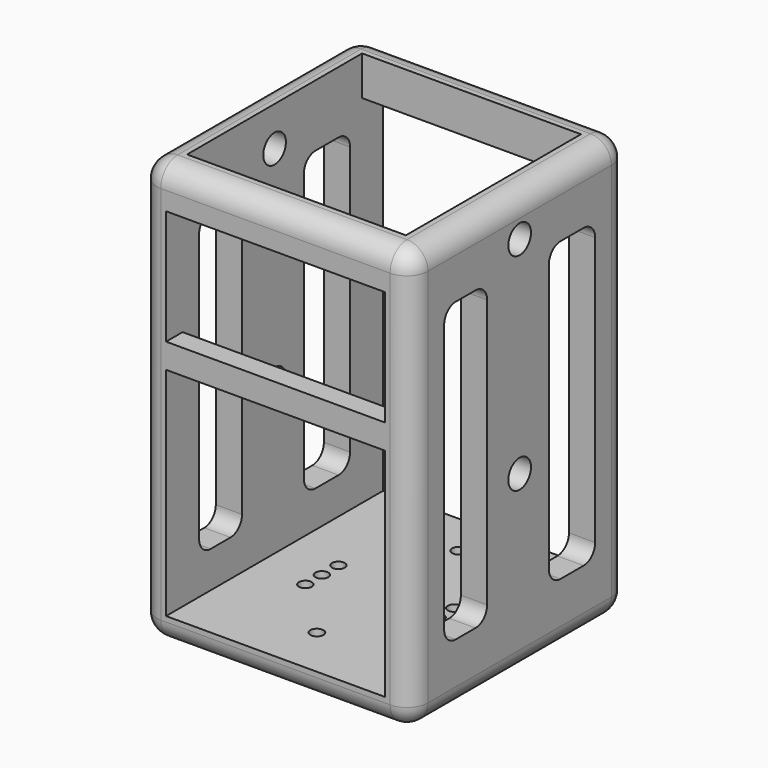
from build123d import *

# Parameters (mm, degrees)
F0_W      = 65.7
F0_H      = 65.7
F1_DEPTH  = 3.175
F2_W      = 65.7
F2_H      = 99
F2_W_2    = 53
F2_H_2    = 86.3
F3_DEPTH  = 65.7
F4_DEPTH  = 6.35
F5_R      = 3.429
F6_DEPTH  = 65.701
F7_R      = 5.08
F8_W      = 53
F8_H      = 6
F9_DEPTH  = 5
F10_R     = 1.5875
F10_R_2   = 1.55
F11_DEPTH = 10


# Not quite as in the source:
# - a length typed as a fraction of an inch, garbled in the dataset ("3 / 203.2 mm" for 3/8 in), is restored


with BuildPart() as f1:
    # F0 (on Top) → F1 (new body)
    with BuildSketch(Plane.XY):
        Rectangle(F0_W, F0_H)
        Polygon((26.5, 26.5), (26.5, -26.5), (-26.5, -26.5), (-26.5, -24.0082931455), (-26.5, 26.5), align=None, mode=Mode.SUBTRACT)
    extrude(amount=F1_DEPTH)

    # F2 (on face) → F3 (join)
    with BuildSketch(Plane.XZ.offset(32.85)):
        with Locations((0, -49.5)):
            Rectangle(F2_W, F2_H)
        with Locations((0, -49.5)):
            Rectangle(F2_W_2, F2_H_2, mode=Mode.SUBTRACT)
    extrude(amount=-F3_DEPTH)

    # F4 (cut): faces of the model
    f4_faces = [f1.faces().sort_by_distance(p)[0] for p in [
        (0, 0, 0),
        (0, 0, 0),
    ]]
    extrude(f4_faces, amount=-F4_DEPTH, mode=Mode.SUBTRACT)

    # F5 (on face) → F6 (cut, through all)
    with BuildSketch(Plane(origin=(-32.85, 0, 0), x_dir=(0, -1, 0), z_dir=(-1, 0, 0))):
        with Locations((0, -56.35)):
            Circle(F5_R)
        with Locations((0, -6.35)):
            Circle(F5_R)
        with BuildLine():
            ThreePointArc((22.85, -15.325), (21.8248737342, -12.8501262658), (19.35, -11.825))
            Line((19.35, -11.825), (13.35, -11.825))
            ThreePointArc((13.35, -11.825), (10.8751262658, -12.8501262658), (9.85, -15.325))
            Line((9.85, -15.325), (9.85, -80.325))
            ThreePointArc((9.85, -80.325), (10.8751262658, -82.7998737342), (13.35, -83.825))
            Line((13.35, -83.825), (19.35, -83.825))
            ThreePointArc((19.35, -83.825), (21.8248737342, -82.7998737342), (22.85, -80.325))
            Line((22.85, -80.325), (22.85, -15.325))
        make_face()
        with BuildLine():
            ThreePointArc((-8.86, -15.325), (-9.8851262658, -12.8501262658), (-12.36, -11.825))
            Line((-12.36, -11.825), (-19.36, -11.825))
            ThreePointArc((-19.36, -11.825), (-21.8348737342, -12.8501262658), (-22.86, -15.325))
            Line((-22.86, -15.325), (-22.86, -80.325))
            ThreePointArc((-22.86, -80.325), (-21.8348737342, -82.7998737342), (-19.36, -83.825))
            Line((-19.36, -83.825), (-12.36, -83.825))
            ThreePointArc((-12.36, -83.825), (-9.8851262658, -82.7998737342), (-8.86, -80.325))
            Line((-8.86, -80.325), (-8.86, -15.325))
        make_face()
    extrude(amount=-F6_DEPTH, mode=Mode.SUBTRACT)

    # F7
    f7_edges = [f1.edges().sort_by_distance(p)[0] for p in [
        (0, -32.85, 3.175),
        (32.85, 0, 3.175),
        (0, 32.85, 3.175),
        (-32.85, 0, 3.175),
        (32.85, 32.85, -47.9125),
        (32.85, -32.85, -47.9125),
        (-32.85, -32.85, -47.9125),
        (-32.85, 32.85, -47.9125),
        (0, 32.85, -99),
        (-32.85, 0, -99),
        (32.85, 0, -99),
        (0, -32.85, -99),
    ]]
    fillet(f7_edges, radius=F7_R)

    # F8 (on face) → F9 (join)
    with BuildSketch(Plane.XZ.offset(32.85)):
        with Locations((0, -37.15)):
            Rectangle(F8_W, F8_H)
    extrude(amount=-F9_DEPTH)

    # F10 (on face) → F11 (cut)
    with BuildSketch(Plane(origin=(0, 0, -99), x_dir=(1, 0, 0), z_dir=(0, 0, -1))):
        with Locations((0, 20.3174948692)):
            Circle(F10_R)
        with Locations((-14.0181705356, 1.279)):
            Circle(F10_R_2)
        with Locations((14.0181705356, 1.279)):
            Circle(F10_R_2)
        with Locations((-14.0181705356, 6.279)):
            Circle(F10_R_2)
        with Locations((-14.0181705356, -3.721)):
            Circle(F10_R_2)
        with Locations((14.0181705356, 6.279)):
            Circle(F10_R_2)
        with Locations((14.0181705356, -3.721)):
            Circle(F10_R_2)
        with Locations((0, -22.6024445146)):
            Circle(F10_R)
    extrude(amount=-F11_DEPTH, mode=Mode.SUBTRACT)


solid = f1.part
